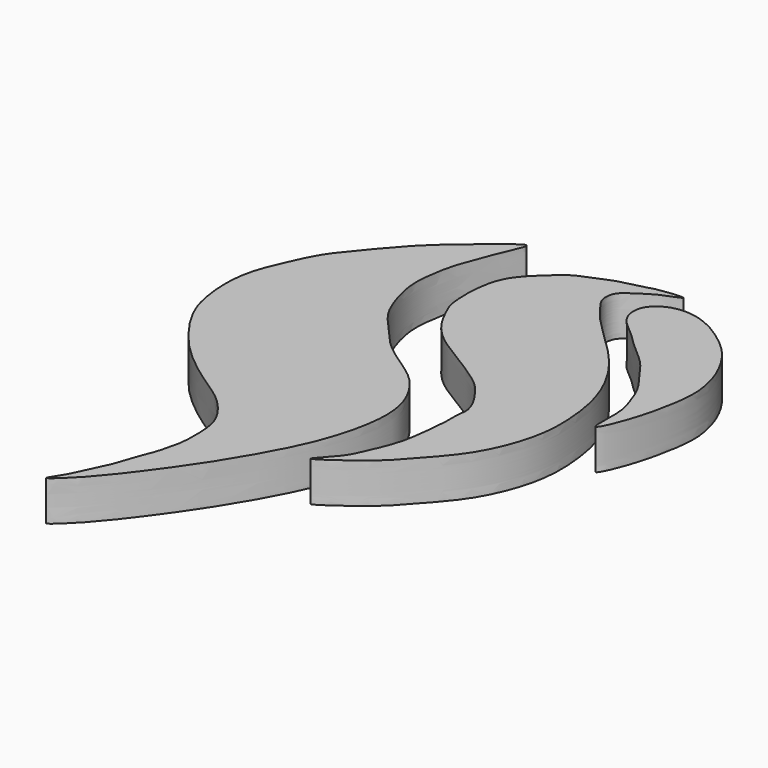
from build123d import *

# Parameters (mm, degrees)
F1_DEPTH = 1


with BuildPart() as f1:
    # F0 (on Top) → F1 (new body)
    with BuildSketch(Plane.XY):
        with BuildLine():
            add(Edge.make_bspline(
                [(-1.7063466899, -8.3813841261), (-1.7172805894, -8.356372089), (-1.4618324448, -8.0039075036), (-1.3486043102, -7.6795461622), (-1.0776562489, -7.2210430398), (-0.8714200389, -6.5104210496), (-0.7621627446, -6.2836676174), (-0.649575152, -5.911187858), (-0.5636515708, -5.5134581403), (-0.559205103, -5.1460177792), (-0.5740627786, -4.5967518997), (-0.7772446868, -4.1487995962), (-1.2028797853, -3.663554963), (-1.666480552, -3.3601936741), (-2.3428107494, -2.9020415747), (-2.9266231473, -2.3917442037), (-3.3466822727, -1.9077255379), (-3.7371733209, -1.3371620596), (-3.9916947354, -0.7967535956), (-4.1301949133, 0.0126345805), (-4.0812160381, 0.8549816194), (-3.7766593231, 1.5750216785), (-3.4377359922, 2.3370550117), (-3.0412151905, 2.8172568258), (-2.6945446606, 3.2376263433), (-2.2568308925, 3.7405256594), (-1.8659526784, 4.1213964081), (-0.9872635587, 4.8454434996), (-0.3591387881, 5.3334781663), (-0.7502789359, 4.5607954862), (-0.830959046, 4.2489388349), (-1.0924788876, 3.6425641002), (-1.1878991132, 3.1579373629), (-1.2804625153, 2.4779935766), (-1.0968094396, 1.7525120592), (-0.8399008925, 1.1371322248), (-0.3301990848, 0.6331857574), (0.0470767825, 0.1284664386), (0.8442647078, -0.3757514409), (1.3488562772, -0.7745775569), (1.8019602117, -1.5432487583), (1.8476062108, -2.4261673064), (1.6399035407, -3.3269010511), (1.3786199936, -4.0719598871), (0.8877681746, -5.0178020423), (0.2853774496, -6.0037904337), (-0.314372701, -6.8405090608), (-1.1049491817, -7.8899227365), (-1.6926217191, -8.4127809286), (-1.7063466899, -8.3813841261)],
                knots=[0, 0, 0, 0, 0.0163169974, 0.0327278235, 0.0517754297, 0.0739875758, 0.0872044526, 0.1030911086, 0.1197117716, 0.1355665758, 0.1545519414, 0.1728424407, 0.193351839, 0.2128621959, 0.2363297764, 0.2593385408, 0.2801969269, 0.3015722385, 0.3216494846, 0.345049995, 0.368856622, 0.3919140301, 0.4156197564, 0.4359924306, 0.4552730101, 0.4760488343, 0.4956379948, 0.5246634953, 0.5420761766, 0.5615275854, 0.5781684767, 0.5985863803, 0.6172109362, 0.6384709023, 0.6609389978, 0.6821460035, 0.7037604549, 0.7246286854, 0.7495312655, 0.7706303931, 0.7945040588, 0.8189155822, 0.8436989189, 0.8668003249, 0.8936026697, 0.9215037646, 0.9480344616, 0.9795178002, 1, 1, 1, 1], degree=3))
        make_face()
    extrude(amount=F1_DEPTH)


with BuildPart() as f1b:
    # F0 (on Top) → F1, piece 2 (new body)
    with BuildSketch(Plane.XY):
        with BuildLine():
            add(Edge.make_bspline(
                [(1.8152594616, -4.5203130499), (1.7943951737, -4.4948404032), (2.2758030447, -4.0287618607), (2.4148522273, -3.6633253349), (2.6089792486, -3.2545033687), (2.7524521188, -2.8367032316), (2.8038665592, -2.5350003668), (2.8526347568, -2.144752812), (2.9053202808, -1.7039101337), (2.8848986467, -1.2727938084), (2.9528130645, -1.0041134884), (2.7851445007, -0.6266828726), (2.5470207986, -0.2944471709), (2.2708993801, 0.0423692032), (1.3076645699, 0.6387658594), (0.6858189927, 1.0109340217), (0.2466710969, 1.4725782511), (0.0098214938, 1.9544465321), (-0.133685069, 2.2630727654), (-0.1631203169, 2.7311951955), (-0.1526234207, 3.1525603082), (-0.0413198376, 3.7334861987), (0.2744146742, 4.1180458062), (0.4969984962, 4.3305652307), (0.8194845164, 4.6270223223), (1.0686315322, 4.781993753), (1.5561727074, 4.9613852635), (1.7854315338, 5.0763663142), (2.3605761147, 5.1882372217), (2.5737944673, 5.2897433674), (3.5043978679, 5.3836337842), (2.873304713, 5.1790124148), (2.5859052879, 5.0092218678), (2.2839074332, 4.8104991946), (2.0431014989, 4.6215452219), (2.0306831516, 4.2458950594), (2.2670553113, 3.9619243992), (2.5858114971, 3.5008483439), (3.7657613954, 2.4688756461), (4.3351302536, 1.5406909889), (4.6380633792, 0.7137311224), (4.7569512853, -0.406620434), (4.6127603553, -1.3200583491), (4.165986691, -2.391136837), (3.3811336055, -3.2379368032), (2.8945895139, -3.8239392806), (1.8438750445, -4.5552490437), (1.8152594616, -4.5203130499)],
                knots=[0, 0, 0, 0, 0.023185984, 0.0439252412, 0.0637554775, 0.083664716, 0.1002557297, 0.1189153585, 0.13927487, 0.1588416442, 0.1743544604, 0.1931703577, 0.2122023718, 0.2320218575, 0.2638176929, 0.2900762529, 0.3136932353, 0.3354447975, 0.3529453641, 0.3730506057, 0.3928972993, 0.4158415535, 0.4366865281, 0.4535992853, 0.4730061564, 0.4898598377, 0.5109170755, 0.5270386601, 0.5489056107, 0.5664139897, 0.5896505899, 0.6071740681, 0.6263394033, 0.6440985832, 0.6602765941, 0.6774919405, 0.6950454963, 0.7174578616, 0.7550491607, 0.7867313399, 0.8146480422, 0.8461267173, 0.8751232737, 0.9073376777, 0.938788797, 0.9682001873, 1, 1, 1, 1], degree=3))
        make_face()
    extrude(amount=F1_DEPTH)


with BuildPart() as f1c:
    # F0 (on Top) → F1, piece 3 (new body)
    with BuildSketch(Plane.XY):
        with BuildLine():
            add(Edge.make_bspline(
                [(5.3081025303, 0.0072720654), (5.358744481, -0.0198924155), (5.6589437736, 0.668307656), (5.8639474128, 1.5221957507), (5.9933526607, 2.389669732), (5.7857829181, 3.2122419875), (5.4253746849, 3.8419065573), (5.0774654447, 4.2147183052), (4.6596310914, 4.5361568296), (4.098860296, 4.8688636077), (3.3577684152, 4.9499326907), (2.7896569721, 4.5424142554), (2.8538286391, 3.915402952), (3.3462454169, 3.5674877076), (3.608241233, 3.2838207929), (3.9373100815, 2.9910724384), (4.3474584446, 2.6432135541), (4.5936707174, 2.2514971418), (4.9842785571, 1.780692297), (5.1845589911, 1.1990778068), (5.3229710803, 0.7746499481), (5.2548770631, 0.0358223516), (5.3081025303, 0.0072720654)],
                knots=[0, 0, 0, 0, 0.0503828158, 0.1150230101, 0.1741090988, 0.2326839764, 0.2868278059, 0.3320139333, 0.3780016046, 0.4296211266, 0.4838662216, 0.5335958108, 0.5801666844, 0.628808414, 0.6686669089, 0.7109264498, 0.7575459333, 0.801183037, 0.8511316083, 0.9000802872, 0.9470468877, 1, 1, 1, 1], degree=3))
        make_face()
    extrude(amount=F1_DEPTH)


solid = Compound([f1.part, f1b.part, f1c.part])
